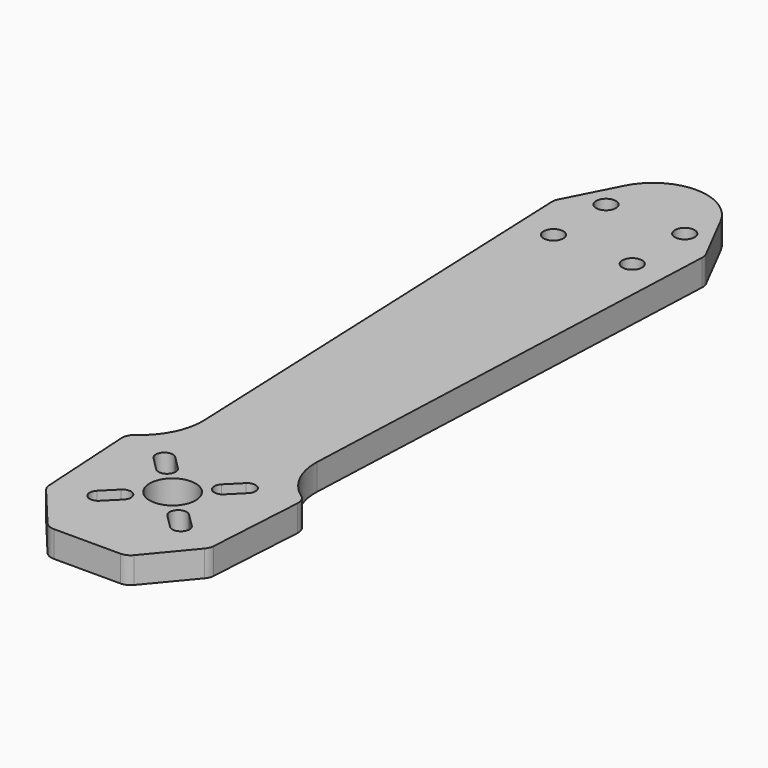
from build123d import *

# Parameters (mm, degrees)
F0_R     = 3.5
F0_R_2   = 1.5
F1_DEPTH = 4
F2_R     = 2


with BuildPart() as f1:
    # F0 (on Top) → F1 (new body)
    with BuildSketch(Plane.XY):
        with BuildLine():
            Line((-12.5, -8.5), (-6, -16.3))
            Line((-6, -16.3), (0, -16.3))
            Line((0, -16.3), (6, -16.3))
            Line((6, -16.3), (12.5, -8.5))
            Line((12.5, -8.5), (13.5, 8.2))
            add(Edge.make_bspline(
                [(8.6, 16.7), (8.4917186517, 14.0737226405), (9.7758937627, 10.1948501542), (13.5, 8.2)],
                knots=[0, 0, 0, 0, 9.8112180691, 9.8112180691, 9.8112180691, 9.8112180691], degree=3))
            Line((8.6, 16.7), (11.5, 87.0371768306))
            Line((11.5, 87.0371768306), (7.3, 95.2371768306))
            ThreePointArc((7.3, 95.2371768306), (0, 99.7), (-7.3, 95.2371768306))
            Line((-7.3, 95.2371768306), (-11.5, 87.0371768306))
            Line((-11.5, 87.0371768306), (-8.6, 16.7))
            add(Edge.make_bspline(
                [(-8.6, 16.7), (-8.4917186517, 14.0737226405), (-9.7758937627, 10.1948501542), (-13.5, 8.2)],
                knots=[0, 0, 0, 0, 9.8112180691, 9.8112180691, 9.8112180691, 9.8112180691], degree=3))
            Line((-13.5, 8.2), (-12.5, -8.5))
        make_face()
        with BuildLine():
            Line((-7.2192388155, -5.3807611845), (-5.1686291501, -3.330151519))
            ThreePointArc((-5.1686291501, -3.330151519), (-3.330151519, -3.330151519), (-3.330151519, -5.1686291501))
            Line((-3.330151519, -5.1686291501), (-5.3807611845, -7.2192388155))
            ThreePointArc((-5.3807611845, -7.2192388155), (-7.2192388155, -7.2192388155), (-7.2192388155, -5.3807611845))
        make_face(mode=Mode.SUBTRACT)
        with BuildLine():
            ThreePointArc((-3.330151519, 5.1686291501), (-3.330151519, 3.330151519), (-5.1686291501, 3.330151519))
            Line((-5.1686291501, 3.330151519), (-7.2192388155, 5.3807611845))
            ThreePointArc((-7.2192388155, 5.3807611845), (-7.2192388155, 7.2192388155), (-5.3807611845, 7.2192388155))
            Line((-5.3807611845, 7.2192388155), (-3.330151519, 5.1686291501))
        make_face(mode=Mode.SUBTRACT)
        with BuildLine():
            Line((5.3807611845, -7.2192388155), (3.330151519, -5.1686291501))
            ThreePointArc((3.330151519, -5.1686291501), (3.330151519, -3.330151519), (5.1686291501, -3.330151519))
            Line((5.1686291501, -3.330151519), (7.2192388155, -5.3807611845))
            ThreePointArc((7.2192388155, -5.3807611845), (7.2192388155, -7.2192388155), (5.3807611845, -7.2192388155))
        make_face(mode=Mode.SUBTRACT)
        Circle(F0_R, mode=Mode.SUBTRACT)
        with BuildLine():
            Line((7.2192388155, 5.3807611845), (5.1686291501, 3.330151519))
            ThreePointArc((5.1686291501, 3.330151519), (3.330151519, 3.330151519), (3.330151519, 5.1686291501))
            Line((3.330151519, 5.1686291501), (5.3807611845, 7.2192388155))
            ThreePointArc((5.3807611845, 7.2192388155), (7.2192388155, 7.2192388155), (7.2192388155, 5.3807611845))
        make_face(mode=Mode.SUBTRACT)
        with Locations((-6, 80.0371768306)):
            Circle(F0_R_2, mode=Mode.SUBTRACT)
        with Locations((-6, 90.0371768306)):
            Circle(F0_R_2, mode=Mode.SUBTRACT)
        with Locations((6, 80.0371768306)):
            Circle(F0_R_2, mode=Mode.SUBTRACT)
        with Locations((6, 90.0371768306)):
            Circle(F0_R_2, mode=Mode.SUBTRACT)
    extrude(amount=F1_DEPTH)

    # F2
    f2_edges = [f1.edges().sort_by_distance(p)[0] for p in [
        (-11.5, 87.037177, 2),
        (11.5, 87.037177, 2),
        (13.5, 8.2, 2),
        (-13.5, 8.2, 2),
        (-12.5, -8.5, 2),
        (12.5, -8.5, 2),
        (6, -16.3, 2),
        (-6, -16.3, 2),
    ]]
    fillet(f2_edges, radius=F2_R)


solid = f1.part
